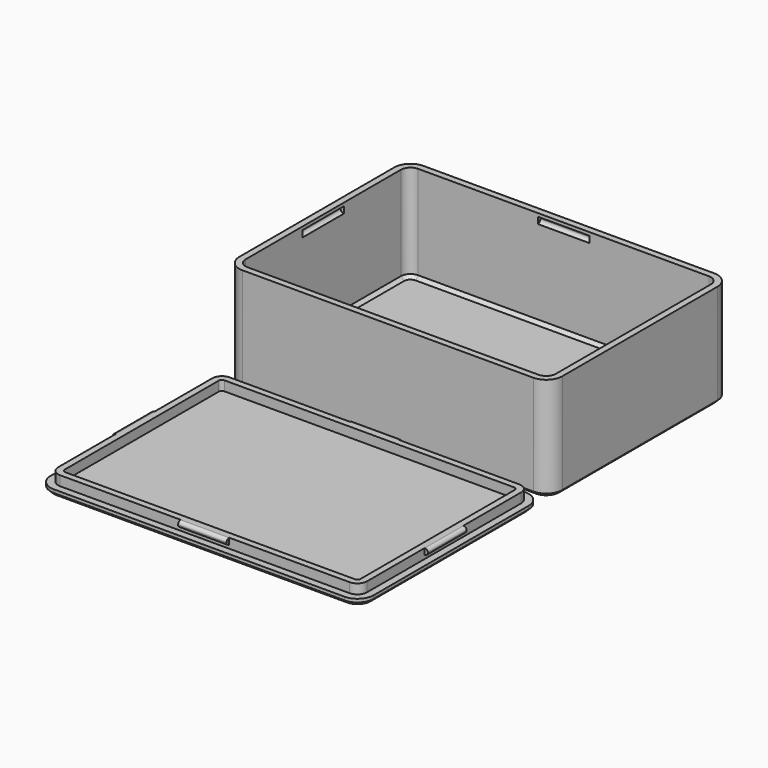
from build123d import *

# Parameters (mm, degrees)
F1_W           = 100
F1_H           = 70
F2_DEPTH       = 2
F3_DEPTH       = 30
F4_R           = 5
F5_T           = -2
F8_DEPTH       = 1
F9_DEPTH       = 1
F11_DEPTH      = 1
F13_DEPTH      = 1
F1_W_2         = 95.6
F1_H_2         = 65.6
F14_DEPTH      = 2
F15_R          = 5
F16_DEPTH      = 3
F17_R          = 3
F18_T          = -2
F20_DEPTH      = 1
F22_DEPTH      = 1
F24_DEPTH      = 1
F26_DEPTH      = 1
F27_F1_R       = 0.9999
F27_F2_R       = 0.9999
F27_F3_R       = 0.9999
F27_F4_R       = 0.9999
F27_F5_R       = 0.9999
F27_F6_R       = 0.9999
F27_F7_R       = 0.9999
F27_F8_R       = 0.9999
F27_2_T1_DEPTH = 20
F27_2_T3_DEPTH = 20
F28_TEXT_SIZE  = 27.7777777778
F29_DEPTH      = 1
F30_SIZE       = 1
F30_2_SIZE     = 1


# Not quite as in the source:
# - a fillet or chamfer that OpenCascade refuses, or shapes differently, is made with other operations: its cross-section is extruded or revolved along the edge and cut away or added
# - a fillet or chamfer is up to 0.001 mm smaller than in the source, because OpenCascade refuses the exact size
# - a feature names something its author has since deleted; it is built from what else it names
# - Text() gives the source's letters only with a copy of the font that has no kerning and outlines rounded to 1/6400 em; it was checked with that copy


with BuildPart() as f2:
    # F1 (on Top) → F2 (new body)
    with BuildSketch(Plane.XY):
        Rectangle(F1_W, F1_H)
    extrude(amount=-F2_DEPTH)

    # F3 (add): a face of the model
    f3_faces = [f2.faces().sort_by_distance(p)[0] for p in [
        (0, 0, 0),
    ]]
    extrude(f3_faces, amount=F3_DEPTH)

    # F4
    f4_edges = [f2.edges().sort_by_distance(p)[0] for p in [
        (-50, 35, 14),
        (-50, -35, 14),
        (50, -35, 14),
        (50, 35, 14),
    ]]
    fillet(f4_edges, radius=F4_R)

    # F5
    f5_openings = [f2.faces().sort_by_distance(p)[0] for p in [
        (0, 0, 30),
    ]]
    offset(amount=F5_T, openings=f5_openings)

    # F7 (on face) → F8 (cut)
    with BuildSketch(Plane.XZ.offset(-33)):
        Polygon((8, 29), (0, 29), (-8, 29), (-8, 27), (8, 27), align=None)
    extrude(amount=-F8_DEPTH, mode=Mode.SUBTRACT)

    # F6 (on face) → F9 (cut)
    with BuildSketch(Plane.YZ.offset(-48)):
        Polygon((8, 29), (0, 29), (-8, 29), (-8, 27), (8, 27), align=None)
    extrude(amount=-F9_DEPTH, mode=Mode.SUBTRACT)

    # F10 (on face) → F11 (cut)
    with BuildSketch(Plane(origin=(0, -33, 0), x_dir=(-1, 0, 0), z_dir=(0, 1, 0))):
        Polygon((8, 29), (0, 29), (-8, 29), (-8, 27), (8, 27), align=None)
    extrude(amount=-F11_DEPTH, mode=Mode.SUBTRACT)

    # F12 (on face) → F13 (cut)
    with BuildSketch(Plane(origin=(48, 0, 0), x_dir=(0, -1, 0), z_dir=(-1, 0, 0))):
        Polygon((8, 29), (0, 29), (-8, 29), (-8, 27), (8, 27), align=None)
    extrude(amount=-F13_DEPTH, mode=Mode.SUBTRACT)

    # F27: fillet of radius 1 on 8 edges, made by hand

    # F27_f1 (radius 1 in the source; OpenCascade refuses exactly that, so slightly less here)
    f27_f1_edges = [f2.edges().sort_by_distance(p)[0] for p in [
        (0, -34, 29),
    ]]
    fillet(f27_f1_edges, radius=F27_F1_R)

    # F27_f2 (radius 1 in the source; OpenCascade refuses exactly that, so slightly less here)
    f27_f2_edges = [f2.edges().sort_by_distance(p)[0] for p in [
        (0, -34, 27),
    ]]
    fillet(f27_f2_edges, radius=F27_F2_R)

    # F27_f3 (radius 1 in the source; OpenCascade refuses exactly that, so slightly less here)
    f27_f3_edges = [f2.edges().sort_by_distance(p)[0] for p in [
        (-49, 0, 29),
    ]]
    fillet(f27_f3_edges, radius=F27_F3_R)

    # F27_f4 (radius 1 in the source; OpenCascade refuses exactly that, so slightly less here)
    f27_f4_edges = [f2.edges().sort_by_distance(p)[0] for p in [
        (-49, 0, 27),
    ]]
    fillet(f27_f4_edges, radius=F27_F4_R)

    # F27_f5 (radius 1 in the source; OpenCascade refuses exactly that, so slightly less here)
    f27_f5_edges = [f2.edges().sort_by_distance(p)[0] for p in [
        (0, 34, 29),
    ]]
    fillet(f27_f5_edges, radius=F27_F5_R)

    # F27_f6 (radius 1 in the source; OpenCascade refuses exactly that, so slightly less here)
    f27_f6_edges = [f2.edges().sort_by_distance(p)[0] for p in [
        (0, 34, 27),
    ]]
    fillet(f27_f6_edges, radius=F27_F6_R)

    # F27_f7 (radius 1 in the source; OpenCascade refuses exactly that, so slightly less here)
    f27_f7_edges = [f2.edges().sort_by_distance(p)[0] for p in [
        (49, 0, 29),
    ]]
    fillet(f27_f7_edges, radius=F27_F7_R)

    # F27_f8 (radius 1 in the source; OpenCascade refuses exactly that, so slightly less here)
    f27_f8_edges = [f2.edges().sort_by_distance(p)[0] for p in [
        (49, 0, 27),
    ]]
    fillet(f27_f8_edges, radius=F27_F8_R)

    # F30
    f30_edges = [f2.edges().sort_by_distance(p)[0] for p in [
        (0, -35, -2),
        (48, 0, 0),
        (47.12132, 32.12132, 0),
        (0, -33, 0),
        (47.12132, -32.12132, 0),
        (0, 33, 0),
        (-47.12132, 32.12132, 0),
        (-48, 0, 0),
        (-47.12132, -32.12132, 0),
        (48.535534, -33.535534, -2),
        (50, 0, -2),
        (48.535534, 33.535534, -2),
        (0, 35, -2),
        (-48.535534, 33.535534, -2),
        (-50, 0, -2),
        (-48.535534, -33.535534, -2),
    ]]
    chamfer(f30_edges, length=F30_SIZE)


with BuildPart() as f14:
    # F1 (on Top) → F14 (new body)
    with BuildSketch(Plane.XY):
        with Locations((0, -73)):
            Rectangle(F1_W, F1_H)
        with Locations((0, -73)):
            Rectangle(F1_W_2, F1_H_2, mode=Mode.SUBTRACT)
        with Locations((0, -73)):
            Rectangle(F1_W_2, F1_H_2)
    extrude(amount=-F14_DEPTH)

    # F15
    f15_edges = [f14.edges().sort_by_distance(p)[0] for p in [
        (-50, -108, -1),
        (-50, -38, -1),
        (50, -108, -1),
        (50, -38, -1),
    ]]
    fillet(f15_edges, radius=F15_R)

    # F1 (on Top) → F16 (join)
    with BuildSketch(Plane.XY):
        with Locations((0, -73)):
            Rectangle(F1_W_2, F1_H_2)
    extrude(amount=F16_DEPTH)

    # F17
    f17_edges = [f14.edges().sort_by_distance(p)[0] for p in [
        (-47.8, -105.8, 1.5),
        (47.8, -105.8, 1.5),
        (47.8, -40.2, 1.5),
        (-47.8, -40.2, 1.5),
    ]]
    fillet(f17_edges, radius=F17_R)

    # F18
    f18_openings = [f14.faces().sort_by_distance(p)[0] for p in [
        (0, -73, 3),
    ]]
    offset(amount=F18_T, openings=f18_openings, kind=Kind.INTERSECTION)

    # F19 (on face) → F20 (join)
    with BuildSketch(Plane.XZ.offset(105.8)):
        Polygon((-7.5, 1.1), (7.5, 1.1), (7.5, 3), (0, 3), (-7.5, 3), align=None)
    extrude(amount=F20_DEPTH)

    # F21 (on face) → F22 (join)
    with BuildSketch(Plane(origin=(-47.8, 0, 0), x_dir=(0, -1, 0), z_dir=(-1, 0, 0))):
        Polygon((65.5, 1.1), (80.5, 1.1), (80.5, 3), (73, 3), (65.5, 3), align=None)
    extrude(amount=F22_DEPTH)

    # F23 (on face) → F24 (join)
    with BuildSketch(Plane.YZ.offset(47.8)):
        Polygon((-80.5, 1.1), (-65.5, 1.1), (-65.5, 3), (-73, 3), (-80.5, 3), align=None)
    extrude(amount=F24_DEPTH)

    # F25 (on face) → F26 (join)
    with BuildSketch(Plane(origin=(0, -40.2, 0), x_dir=(-1, 0, 0), z_dir=(0, 1, 0))):
        Polygon((-7.5, 1.1), (7.5, 1.1), (7.5, 3), (0, 3), (-7.5, 3), align=None)
    extrude(amount=F26_DEPTH)

    # F27#2: fillet of radius 1 on 8 edges, made by hand

    # F27_2_s2 → F27_2_t1 (cut)
    with BuildSketch(Plane.YZ.offset(-10)):
        with BuildLine():
            ThreePointArc((-40.2, 3), (-39.4928932188, 2.7071067812), (-39.2, 2))
            Line((-39.2, 2), (-39.2, 3))
            Line((-39.2, 3), (-40.2, 3))
        make_face()
        with BuildLine():
            ThreePointArc((-40.2, 1.1), (-39.4928932188, 1.3928932188), (-39.2, 2.1))
            Line((-39.2, 2.1), (-39.2, 1.1))
            Line((-39.2, 1.1), (-40.2, 1.1))
        make_face()
        with BuildLine():
            ThreePointArc((-105.8, 1.1), (-106.5071067812, 1.3928932188), (-106.8, 2.1))
            Line((-106.8, 2.1), (-106.8, 1.1))
            Line((-106.8, 1.1), (-105.8, 1.1))
        make_face()
        with BuildLine():
            ThreePointArc((-105.8, 3), (-106.5071067812, 2.7071067812), (-106.8, 2))
            Line((-106.8, 2), (-106.8, 3))
            Line((-106.8, 3), (-105.8, 3))
        make_face()
    extrude(amount=F27_2_T1_DEPTH, mode=Mode.SUBTRACT)

    # F27_2_s4 → F27_2_t3 (cut)
    with BuildSketch(Plane.XZ.offset(63)):
        with BuildLine():
            ThreePointArc((47.8, 1.1), (48.5071067812, 1.3928932188), (48.8, 2.1))
            Line((48.8, 2.1), (48.8, 1.1))
            Line((48.8, 1.1), (47.8, 1.1))
        make_face()
        with BuildLine():
            ThreePointArc((47.8, 3), (48.5071067812, 2.7071067812), (48.8, 2))
            Line((48.8, 2), (48.8, 3))
            Line((48.8, 3), (47.8, 3))
        make_face()
        with BuildLine():
            ThreePointArc((-47.8, 1.1), (-48.5071067812, 1.3928932188), (-48.8, 2.1))
            Line((-48.8, 2.1), (-48.8, 1.1))
            Line((-48.8, 1.1), (-47.8, 1.1))
        make_face()
        with BuildLine():
            ThreePointArc((-47.8, 3), (-48.5071067812, 2.7071067812), (-48.8, 2))
            Line((-48.8, 2), (-48.8, 3))
            Line((-48.8, 3), (-47.8, 3))
        make_face()
    extrude(amount=F27_2_T3_DEPTH, mode=Mode.SUBTRACT)

    # F28 (on face) → F29 (cut)
    with BuildSketch(Plane(origin=(0, 0, -2), x_dir=(1, 0, 0), z_dir=(0, 0, -1))):
        with Locations((-39.1473907441, 73.8328003601)):
            Text('neon', F28_TEXT_SIZE, font='Open Sans', text_align=(TextAlign.LEFT, TextAlign.BOTTOM))
        with Locations((-39.1473907441, 46.4856661676)):
            Text('show', F28_TEXT_SIZE, font='Open Sans', text_align=(TextAlign.LEFT, TextAlign.BOTTOM))
    extrude(amount=-F29_DEPTH, mode=Mode.SUBTRACT)

    # F30#2
    f30_2_edges = [f14.edges().sort_by_distance(p)[0] for p in [
        (0, -108, -2),
        (-48.535534, -106.535534, -2),
        (48.535534, -106.535534, -2),
        (-50, -73, -2),
        (50, -73, -2),
        (-48.535534, -39.464466, -2),
        (48.535534, -39.464466, -2),
        (0, -38, -2),
    ]]
    chamfer(f30_2_edges, length=F30_2_SIZE)


solid = Compound([f2.part, f14.part])
